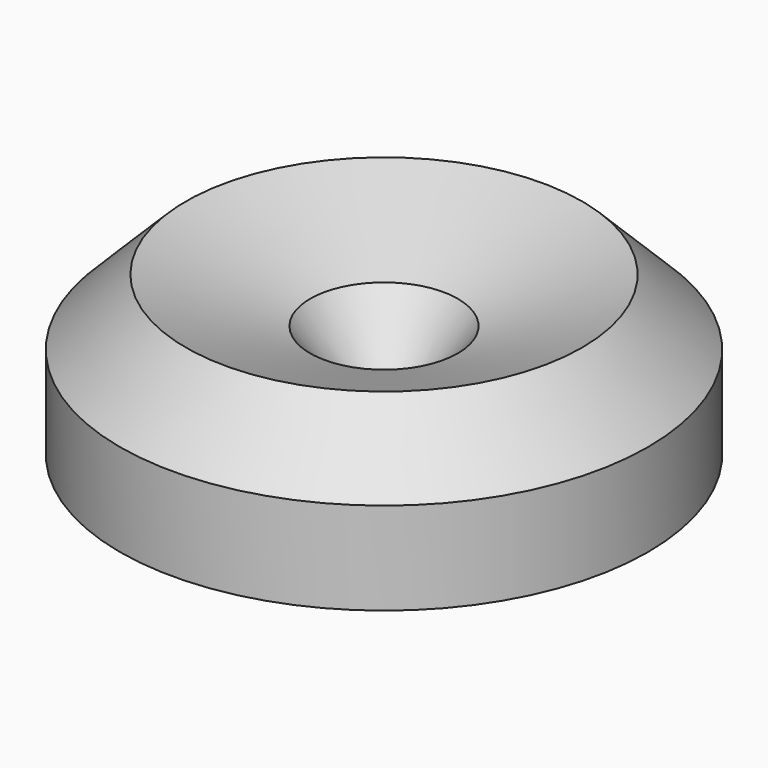
from build123d import *

# Parameters (mm, degrees)
F2_SIZE = 4.99999


# Not quite as in the source:
# - a fillet or chamfer is up to 0.001 mm smaller than in the source, because OpenCascade refuses the exact size


with BuildPart() as f1:
    # F0 (on Front) → F1 (revolve)
    with BuildSketch(Plane.XZ):
        Polygon((0, 1.309961197), (0, 0), (20, 0), (20, 12), (15, 12), (5.5938020571, 8.5615739226), align=None)
    revolve(axis=Axis((0, 0, 0.6549805985), (0, 0, -1)))

    # F2 (size 5 in the source; OpenCascade refuses exactly that, so slightly less here)
    f2_edges = [f1.edges().sort_by_distance(p)[0] for p in [
        (-20, 0, 12),
    ]]
    chamfer(f2_edges, length=F2_SIZE)


solid = f1.part
